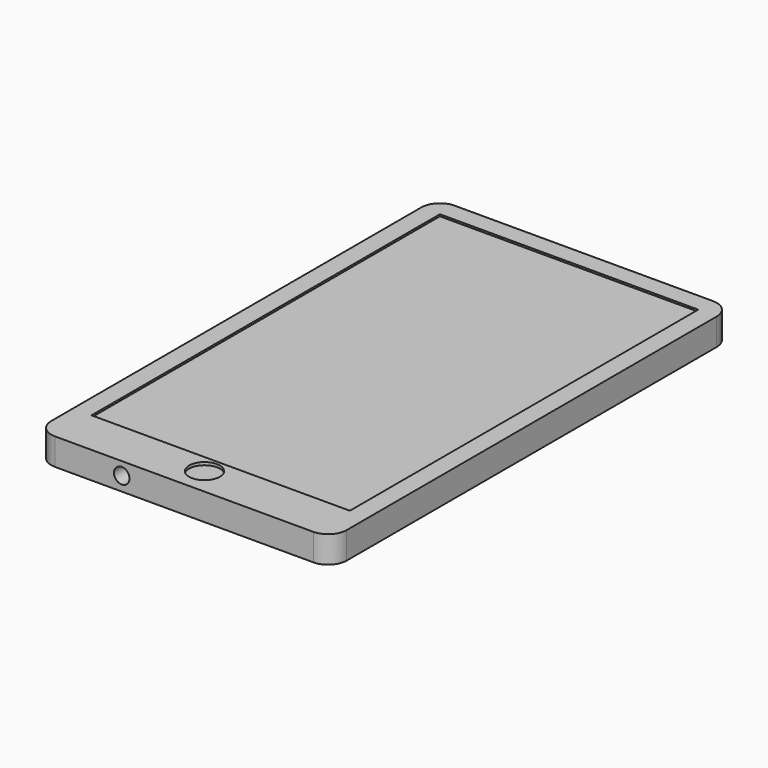
from build123d import *

# Parameters (mm, degrees)
F0_W      = 80.9689760208
F0_H      = 136.9662135839
F1_DEPTH  = 7.366
F2_R      = 5.08
F3_W      = 70.8160358799
F3_H      = 119.3651366365
F4_DEPTH  = 0.508
F5_R      = 4.2062537649
F6_DEPTH  = 0.762
F7_W      = 9.7111202776
F7_H      = 2.8320385609
F8_DEPTH  = 2.54
F9_R      = 2.3153657449
F10_DEPTH = 1.6256
F11_R     = 2.4503430009
F12_DEPTH = 1.778
F14_R     = 3.8927406251
F15_DEPTH = 1.524
F16_R     = 1.7892494252
F17_DEPTH = 4.064
F18_R     = 0.6717284453
F19_DEPTH = 5.08
F21_DEPTH = 3.302
F22_R     = 2.1300534038
F23_DEPTH = 6.858


with BuildPart() as f1:
    # F0 (on Top) → F1 (new body)
    with BuildSketch(Plane.XY):
        with Locations((0.3460086882, -4.4899731874)):
            Rectangle(F0_W, F0_H)
    extrude(amount=F1_DEPTH)

    # F2
    f2_edges = [f1.edges().sort_by_distance(p)[0] for p in [
        (-40.138479, 63.993134, 3.683),
        (40.830497, 63.993134, 3.683),
        (40.830497, -72.97308, 3.683),
        (-40.138479, -72.97308, 3.683),
    ]]
    fillet(f2_edges, radius=F2_R)

    # F3 (on face) → F4 (cut)
    with BuildSketch(Plane.XY.offset(7.366)):
        with Locations((0.3495386177, -0.7694347137)):
            Rectangle(F3_W, F3_H)
    extrude(amount=-F4_DEPTH, mode=Mode.SUBTRACT)

    # F5 (on face) → F6 (cut)
    with BuildSketch(Plane.XY.offset(7.366)):
        with Locations((0, -65.5538588762)):
            Circle(F5_R)
    extrude(amount=-F6_DEPTH, mode=Mode.SUBTRACT)

    # F7 (on face) → F8 (cut)
    with BuildSketch(Plane(origin=(-40.1384793222, 0, 0), x_dir=(0, -1, 0), z_dir=(-1, 0, 0))):
        with Locations((-42.3318911344, 3.4466114594)):
            Rectangle(F7_W, F7_H)
    extrude(amount=-F8_DEPTH, mode=Mode.SUBTRACT)

    # F9 (on face) → F10 (join)
    with BuildSketch(Plane(origin=(-40.1384793222, 0, 0), x_dir=(0, -1, 0), z_dir=(-1, 0, 0))):
        with Locations((-31.1954244971, 3.375432454)):
            Circle(F9_R)
    extrude(amount=F10_DEPTH)

    # F11 (on face) → F12 (join)
    with BuildSketch(Plane(origin=(-40.1384793222, 0, 0), x_dir=(0, -1, 0), z_dir=(-1, 0, 0))):
        with Locations((-22.7978900075, 3.2298590522)):
            Circle(F11_R)
    extrude(amount=F12_DEPTH)

    # F14 (on face) → F15 (cut)
    with BuildSketch(Plane(origin=(0, 0, 0), x_dir=(1, 0, 0), z_dir=(0, 0, -1))):
        with Locations((31.0994051397, -53.9800077677)):
            Circle(F14_R)
    extrude(amount=-F15_DEPTH, mode=Mode.SUBTRACT)

    # F16 (on face) → F17 (cut)
    with BuildSketch(Plane(origin=(0, 0, 0), x_dir=(1, 0, 0), z_dir=(0, 0, -1))):
        with Locations((31.2404166907, -54.5385442674)):
            Circle(F16_R)
    extrude(amount=-F17_DEPTH, mode=Mode.SUBTRACT)

    # F18 (on face) → F19 (cut)
    with BuildSketch(Plane(origin=(0, 0, 0), x_dir=(1, 0, 0), z_dir=(0, 0, -1))):
        with Locations((24.6018432081, -55.6784830987)):
            Circle(F18_R)
    extrude(amount=-F19_DEPTH, mode=Mode.SUBTRACT)

    # F20 (on face) → F21 (cut)
    with BuildSketch(Plane(origin=(0, 0, 0), x_dir=(1, 0, 0), z_dir=(0, 0, -1))):
        with BuildLine():
            add(Edge.make_bspline(
                [(21.838599816, -57.1239739656), (22.3255501081, -55.7146974508), (22.4935564689, -52.3704464682), (19.2282519734, -51.1257918433), (17.6040761183, -53.0174394253), (17.5519956723, -57.9087722175), (20.2838683925, -59.75590869), (21.4647452863, -58.2059415034), (21.838599816, -57.1239739656)],
                knots=[0, 0, 0, 0, 0.2013997834, 0.354787719, 0.491355532, 0.6980279839, 0.8453759603, 1, 1, 1, 1], degree=3))
        make_face()
    extrude(amount=-F21_DEPTH, mode=Mode.SUBTRACT)

    # F22 (on face) → F23 (cut)
    with BuildSketch(Plane.XZ.offset(72.9730799794)):
        with Locations((-16.7610161006, 3.8362841588)):
            Circle(F22_R)
    extrude(amount=-F23_DEPTH, mode=Mode.SUBTRACT)


solid = f1.part
